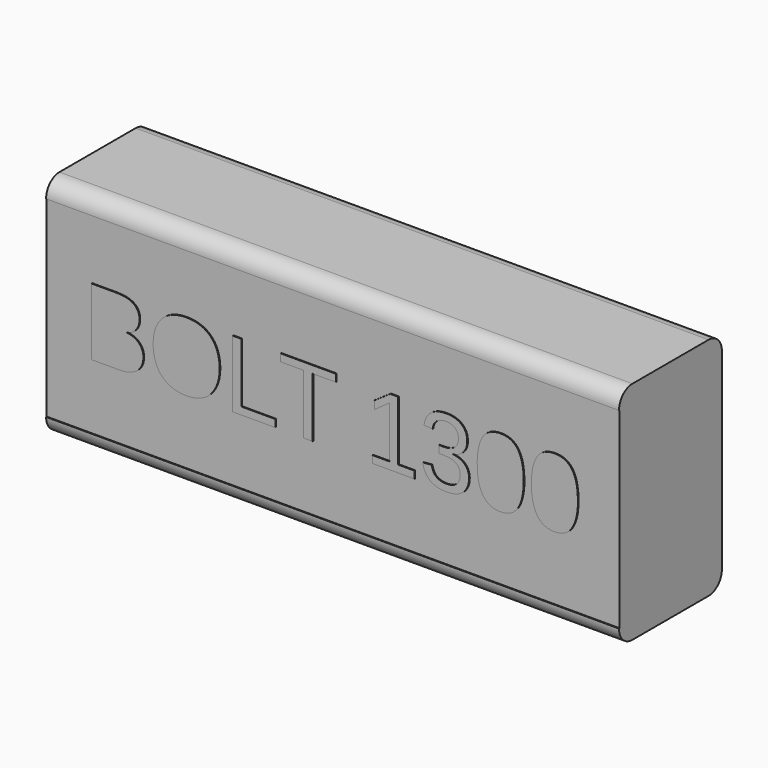
from build123d import *

# Parameters (mm, degrees)
F0_W     = 87.122
F0_H     = 34.29
F1_DEPTH = 9.779
F2_R     = 2.54
F3_W     = 87.122
F3_H     = 29.21
F4_DEPTH = 0.127


with BuildPart() as f1:
    # F0 (on Front) → F1 (new body, symmetric)
    with BuildSketch(Plane.XZ):
        Rectangle(F0_W, F0_H)
    extrude(amount=F1_DEPTH, both=True)

    # F2
    f2_edges = [f1.edges().sort_by_distance(p)[0] for p in [
        (0, 9.779, 17.145),
        (0, 9.779, -17.145),
        (0, -9.779, 17.145),
        (0, -9.779, -17.145),
    ]]
    fillet(f2_edges, radius=F2_R)

    # F3 (on face) → F4 (cut)
    with BuildSketch(Plane.XZ.offset(9.779)):
        Rectangle(F3_W, F3_H)
        with BuildLine():
            add(Edge.make_bspline(
                [(-29.4201796663, -0.1257045448), (-28.7628641118, -0.7945925563), (-28.7628641118, -1.8129687674)],
                knots=[0, 0, 0, 1, 1, 1], degree=2))
            add(Edge.make_bspline(
                [(-28.7628641118, -1.8129687674), (-28.7628641118, -3.1738897042), (-29.7534664263, -3.9295711427)],
                knots=[0, 0, 0, 1, 1, 1], degree=2))
            add(Edge.make_bspline(
                [(-29.7534664263, -3.9295711427), (-30.7440687408, -4.6852525812), (-32.5077111792, -4.6852525812)],
                knots=[0, 0, 0, 1, 1, 1], degree=2))
            Line((-32.5077111792, -4.6852525812), (-36.6460217827, -4.6852525812))
            Line((-36.6460217827, -4.6852525812), (-36.6460217827, 5.5054530046))
            Line((-36.6460217827, 5.5054530046), (-32.9428355603, 5.5054530046))
            add(Edge.make_bspline(
                [(-32.9428355603, 5.5054530046), (-29.3553739074, 5.5054530046), (-29.3553739074, 3.0312617097)],
                knots=[0, 0, 0, 1, 1, 1], degree=2))
            add(Edge.make_bspline(
                [(-29.3553739074, 3.0312617097), (-29.3553739074, 2.128610068), (-29.8610902759, 1.5141126043)],
                knots=[0, 0, 0, 1, 1, 1], degree=2))
            add(Edge.make_bspline(
                [(-29.8610902759, 1.5141126043), (-30.3668066444, 0.8996151405), (-31.2926032, 0.6889964241)],
                knots=[0, 0, 0, 1, 1, 1], degree=2))
            add(Edge.make_bspline(
                [(-31.2926032, 0.6889964241), (-30.0774952208, 0.5431834666), (-29.4201796663, -0.1257045448)],
                knots=[0, 0, 0, 1, 1, 1], degree=2))
        make_face(mode=Mode.SUBTRACT)
        with BuildLine():
            add(Edge.make_bspline(
                [(-17.7713445055, 3.2418804261), (-17.1672622529, 2.0638043091), (-17.1672622529, 0.4575472852)],
                knots=[0, 0, 0, 1, 1, 1], degree=2))
            add(Edge.make_bspline(
                [(-17.1672622529, 0.4575472852), (-17.1672622529, -1.1417662646), (-17.7782879796, -2.3418300498)],
                knots=[0, 0, 0, 1, 1, 1], degree=2))
            add(Edge.make_bspline(
                [(-17.7782879796, -2.3418300498), (-18.3893137063, -3.541893835), (-19.5326724525, -4.1864796868)],
                knots=[0, 0, 0, 1, 1, 1], degree=2))
            add(Edge.make_bspline(
                [(-19.5326724525, -4.1864796868), (-20.6760311986, -4.8310655387), (-22.2313694121, -4.8310655387)],
                knots=[0, 0, 0, 1, 1, 1], degree=2))
            add(Edge.make_bspline(
                [(-22.2313694121, -4.8310655387), (-23.8005945738, -4.8310655387), (-24.9393243372, -4.193423161)],
                knots=[0, 0, 0, 1, 1, 1], degree=2))
            add(Edge.make_bspline(
                [(-24.9393243372, -4.193423161), (-26.0780541006, -3.5557807833), (-26.678664616, -2.3522452611)],
                knots=[0, 0, 0, 1, 1, 1], degree=2))
            add(Edge.make_bspline(
                [(-26.678664616, -2.3522452611), (-27.2792751315, -1.1487097388), (-27.2792751315, 0.4575472852)],
                knots=[0, 0, 0, 1, 1, 1], degree=2))
            add(Edge.make_bspline(
                [(-27.2792751315, 0.4575472852), (-27.2792751315, 2.901650192), (-25.9414991086, 4.2799298141)],
                knots=[0, 0, 0, 1, 1, 1], degree=2))
            add(Edge.make_bspline(
                [(-25.9414991086, 4.2799298141), (-24.6037230858, 5.6582094363), (-22.2151679723, 5.6582094363)],
                knots=[0, 0, 0, 1, 1, 1], degree=2))
            add(Edge.make_bspline(
                [(-22.2151679723, 5.6582094363), (-20.6598297589, 5.6582094363), (-19.5176282585, 5.0390829897)],
                knots=[0, 0, 0, 1, 1, 1], degree=2))
            add(Edge.make_bspline(
                [(-19.5176282585, 5.0390829897), (-18.375426758, 4.4199565431), (-17.7713445055, 3.2418804261)],
                knots=[0, 0, 0, 1, 1, 1], degree=2))
        make_face(mode=Mode.SUBTRACT)
        Polygon((-8.7124252089, -4.6852525812), (-15.2439199087, -4.6852525812), (-15.2439199087, 5.5054530046), (-13.8621685494, 5.5054530046), (-13.8621685494, -3.5557807833), (-8.7124252089, -3.5557807833), align=None, mode=Mode.SUBTRACT)
        Polygon((0.4876780624, 4.3782956981), (-3.0141474092, 4.3782956981), (-3.0141474092, -4.6852525812), (-4.3889552943, -4.6852525812), (-4.3889552943, 4.3782956981), (-7.8884662744, 4.3782956981), (-7.8884662744, 5.5054530046), (0.4876780624, 5.5054530046), align=None, mode=Mode.SUBTRACT)
        Polygon((12.4559130349, -4.6852525812), (6.0702312926, -4.6852525812), (6.0702312926, -3.5789256972), (8.6647761397, -3.5789256972), (8.6647761397, 4.2625711287), (6.3664861904, 2.6192822425), (6.3664861904, 3.8505916615), (8.773557235, 5.5054530046), (9.9747782659, 5.5054530046), (9.9747782659, -3.5789256972), (12.4559130349, -3.5789256972), align=None, mode=Mode.SUBTRACT)
        with BuildLine():
            add(Edge.make_bspline(
                [(20.1284519894, -0.2506870799), (20.7649371214, -0.894115686), (20.7649371214, -1.8708310521)],
                knots=[0, 0, 0, 1, 1, 1], degree=2))
            add(Edge.make_bspline(
                [(20.7649371214, -1.8708310521), (20.7649371214, -3.2826707994), (19.8680717081, -4.0568681691)],
                knots=[0, 0, 0, 1, 1, 1], degree=2))
            add(Edge.make_bspline(
                [(19.8680717081, -4.0568681691), (18.9712062949, -4.8310655387), (17.3070869862, -4.8310655387)],
                knots=[0, 0, 0, 1, 1, 1], degree=2))
            add(Edge.make_bspline(
                [(17.3070869862, -4.8310655387), (15.7610067384, -4.8310655387), (14.8386819198, -4.1320891392)],
                knots=[0, 0, 0, 1, 1, 1], degree=2))
            add(Edge.make_bspline(
                [(14.8386819198, -4.1320891392), (13.9163571013, -3.4331127397), (13.7427702471, -2.0675628202)],
                knots=[0, 0, 0, 1, 1, 1], degree=2))
            Line((13.7427702471, -2.0675628202), (15.0874897442, -1.9448947766))
            add(Edge.make_bspline(
                [(15.0874897442, -1.9448947766), (15.3490272711, -3.7525125514), (17.3070869862, -3.7525125514)],
                knots=[0, 0, 0, 1, 1, 1], degree=2))
            add(Edge.make_bspline(
                [(17.3070869862, -3.7525125514), (18.2907458265, -3.7525125514), (18.8520099884, -3.2676266054)],
                knots=[0, 0, 0, 1, 1, 1], degree=2))
            add(Edge.make_bspline(
                [(18.8520099884, -3.2676266054), (19.4132741502, -2.7827406594), (19.4132741502, -1.8291702071)],
                knots=[0, 0, 0, 1, 1, 1], degree=2))
            add(Edge.make_bspline(
                [(19.4132741502, -1.8291702071), (19.4132741502, -0.9959533071), (18.7733172811, -0.5295832922)],
                knots=[0, 0, 0, 1, 1, 1], degree=2))
            add(Edge.make_bspline(
                [(18.7733172811, -0.5295832922), (18.1333604121, -0.0632132773), (16.925195907, -0.0632132773)],
                knots=[0, 0, 0, 1, 1, 1], degree=2))
            Line((16.925195907, -0.0632132773), (16.1868731539, -0.0632132773))
            Line((16.1868731539, -0.0632132773), (16.1868731539, 1.0639440291))
            Line((16.1868731539, 1.0639440291), (16.895107519, 1.0639440291))
            add(Edge.make_bspline(
                [(16.895107519, 1.0639440291), (17.9667170321, 1.0639440291), (18.5557550906, 1.5314712897)],
                knots=[0, 0, 0, 1, 1, 1], degree=2))
            add(Edge.make_bspline(
                [(18.5557550906, 1.5314712897), (19.1447931491, 1.9989985503), (19.1447931491, 2.8229574847)],
                knots=[0, 0, 0, 1, 1, 1], degree=2))
            add(Edge.make_bspline(
                [(19.1447931491, 2.8229574847), (19.1447931491, 3.6399729451), (18.6645361859, 4.1132864341)],
                knots=[0, 0, 0, 1, 1, 1], degree=2))
            add(Edge.make_bspline(
                [(18.6645361859, 4.1132864341), (18.1842792226, 4.5865999232), (17.2353377531, 4.5865999232)],
                knots=[0, 0, 0, 1, 1, 1], degree=2))
            add(Edge.make_bspline(
                [(17.2353377531, 4.5865999232), (16.3743469564, 4.5865999232), (15.8431711827, 4.1456893136)],
                knots=[0, 0, 0, 1, 1, 1], degree=2))
            add(Edge.make_bspline(
                [(15.8431711827, 4.1456893136), (15.3119954089, 3.7047787039), (15.2240447361, 2.901650192)],
                knots=[0, 0, 0, 1, 1, 1], degree=2))
            Line((15.2240447361, 2.901650192), (13.9163571013, 3.0034878131))
            add(Edge.make_bspline(
                [(13.9163571013, 3.0034878131), (14.0598555674, 4.2556276545), (14.9532492436, 4.9569185454)],
                knots=[0, 0, 0, 1, 1, 1], degree=2))
            add(Edge.make_bspline(
                [(14.9532492436, 4.9569185454), (15.8466429197, 5.6582094363), (17.2492247015, 5.6582094363)],
                knots=[0, 0, 0, 1, 1, 1], degree=2))
            add(Edge.make_bspline(
                [(17.2492247015, 5.6582094363), (18.7837324924, 5.6582094363), (19.6331508322, 4.9453460885)],
                knots=[0, 0, 0, 1, 1, 1], degree=2))
            add(Edge.make_bspline(
                [(19.6331508322, 4.9453460885), (20.4825691719, 4.2324827406), (20.4825691719, 2.9595124767)],
                knots=[0, 0, 0, 1, 1, 1], degree=2))
            add(Edge.make_bspline(
                [(20.4825691719, 2.9595124767), (20.4825691719, 1.9827971105), (19.9363492041, 1.3717713838)],
                knots=[0, 0, 0, 1, 1, 1], degree=2))
            add(Edge.make_bspline(
                [(19.9363492041, 1.3717713838), (19.3901292363, 0.7607456571), (18.3486081113, 0.5431834666)],
                knots=[0, 0, 0, 1, 1, 1], degree=2))
            Line((18.3486081113, 0.5431834666), (18.3486081113, 0.5154095699))
            add(Edge.make_bspline(
                [(18.3486081113, 0.5154095699), (19.4919668574, 0.3927415263), (20.1284519894, -0.2506870799)],
                knots=[0, 0, 0, 1, 1, 1], degree=2))
        make_face(mode=Mode.SUBTRACT)
        with BuildLine():
            add(Edge.make_bspline(
                [(28.2175993939, 4.3343203618), (29.0739612079, 3.0104312872), (29.0739612079, 0.4135719488)],
                knots=[0, 0, 0, 1, 1, 1], degree=2))
            add(Edge.make_bspline(
                [(29.0739612079, 0.4135719488), (29.0739612079, -2.1393120533), (28.1736240576, -3.485188796)],
                knots=[0, 0, 0, 1, 1, 1], degree=2))
            add(Edge.make_bspline(
                [(28.1736240576, -3.485188796), (27.2732869072, -4.8310655387), (25.516587943, -4.8310655387)],
                knots=[0, 0, 0, 1, 1, 1], degree=2))
            add(Edge.make_bspline(
                [(25.516587943, -4.8310655387), (23.7598889787, -4.8310655387), (22.8769105138, -3.4921322701)],
                knots=[0, 0, 0, 1, 1, 1], degree=2))
            add(Edge.make_bspline(
                [(22.8769105138, -3.4921322701), (21.9939320489, -2.1531990016), (21.9939320489, 0.4135719488)],
                knots=[0, 0, 0, 1, 1, 1], degree=2))
            add(Edge.make_bspline(
                [(21.9939320489, 0.4135719488), (21.9939320489, 3.0405196753), (22.8514511086, 4.3493645558)],
                knots=[0, 0, 0, 1, 1, 1], degree=2))
            add(Edge.make_bspline(
                [(22.8514511086, 4.3493645558), (23.7089701682, 5.6582094363), (25.5605632794, 5.6582094363)],
                knots=[0, 0, 0, 1, 1, 1], degree=2))
            add(Edge.make_bspline(
                [(25.5605632794, 5.6582094363), (27.36123758, 5.6582094363), (28.2175993939, 4.3343203618)],
                knots=[0, 0, 0, 1, 1, 1], degree=2))
        make_face(mode=Mode.SUBTRACT)
        with BuildLine():
            add(Edge.make_bspline(
                [(36.4548742474, 4.3343203618), (37.3112360613, 3.0104312872), (37.3112360613, 0.4135719488)],
                knots=[0, 0, 0, 1, 1, 1], degree=2))
            add(Edge.make_bspline(
                [(37.3112360613, 0.4135719488), (37.3112360613, -2.1393120533), (36.410898911, -3.485188796)],
                knots=[0, 0, 0, 1, 1, 1], degree=2))
            add(Edge.make_bspline(
                [(36.410898911, -3.485188796), (35.5105617607, -4.8310655387), (33.7538627964, -4.8310655387)],
                knots=[0, 0, 0, 1, 1, 1], degree=2))
            add(Edge.make_bspline(
                [(33.7538627964, -4.8310655387), (31.9971638322, -4.8310655387), (31.1141853673, -3.4921322701)],
                knots=[0, 0, 0, 1, 1, 1], degree=2))
            add(Edge.make_bspline(
                [(31.1141853673, -3.4921322701), (30.2312069024, -2.1531990016), (30.2312069024, 0.4135719488)],
                knots=[0, 0, 0, 1, 1, 1], degree=2))
            add(Edge.make_bspline(
                [(30.2312069024, 0.4135719488), (30.2312069024, 3.0405196753), (31.088725962, 4.3493645558)],
                knots=[0, 0, 0, 1, 1, 1], degree=2))
            add(Edge.make_bspline(
                [(31.088725962, 4.3493645558), (31.9462450216, 5.6582094363), (33.7978381328, 5.6582094363)],
                knots=[0, 0, 0, 1, 1, 1], degree=2))
            add(Edge.make_bspline(
                [(33.7978381328, 5.6582094363), (35.5985124335, 5.6582094363), (36.4548742474, 4.3343203618)],
                knots=[0, 0, 0, 1, 1, 1], degree=2))
        make_face(mode=Mode.SUBTRACT)
    extrude(amount=-F4_DEPTH, mode=Mode.SUBTRACT)


solid = f1.part
